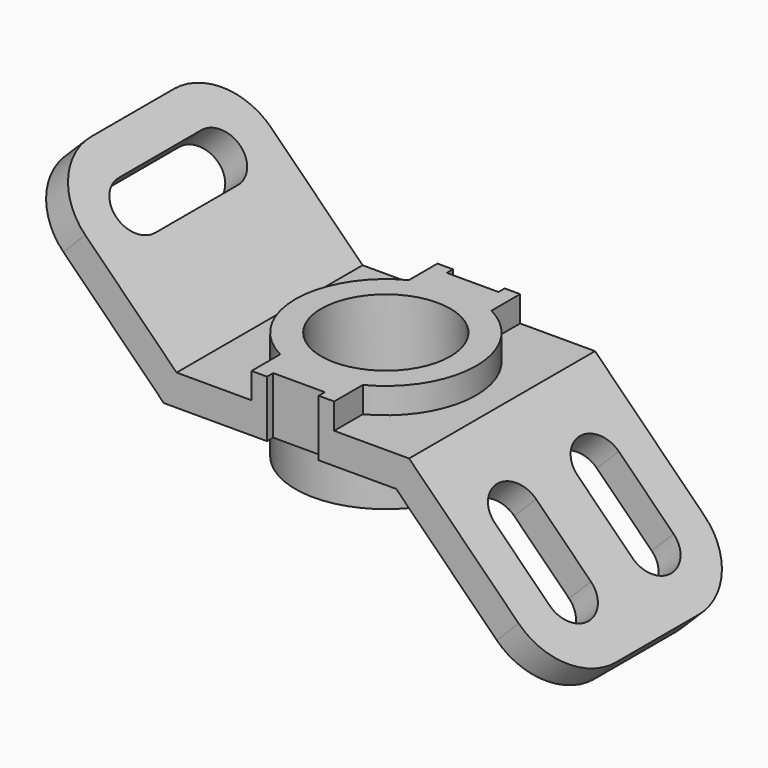
from build123d import *

# Parameters (mm, degrees)
F1_DEPTH       = 45
F2_R           = 35
F3_DEPTH       = 10
F4_R           = 35
F5_DEPTH       = 20
F9_D           = 25
F9_CBORE_D     = 50
F9_CBORE_DEPTH = 32
F10_W          = 20
F10_H          = 3
F11_DEPTH      = 78.5903577751
F12_R          = 25
F14_DEPTH      = 12
F16_DEPTH      = 12


# Not quite as in the source:
# - a pattern or mirror of a feature is missing from the dataset's text; its kind, count and spacing are read off the source's solid


with BuildPart() as f1:
    # F0 (on Front) → F1 (new body, symmetric)
    with BuildSketch(Plane.XZ):
        Polygon((-45, 0), (-98.033008589, 53.033008589), (-106.5182899632, 44.5477272148), (-49.9705627485, -12), (40.0294372515, -12), (96.6187950266, -68.5893577751), (105.1040764009, -60.1040764009), (45, 0), align=None)
    extrude(amount=F1_DEPTH, both=True)

    # F2 (on face) → F3 (join)
    with BuildSketch(Plane.XY):
        Circle(F2_R)
    extrude(amount=F3_DEPTH)

    # F4 (on face) → F5 (join)
    with BuildSketch(Plane(origin=(0, 0, -12), x_dir=(1, 0, 0), z_dir=(0, 0, -1))):
        Circle(F4_R)
    extrude(amount=F5_DEPTH)

    # F6 (on face) → F7 (join, up to the next surface of F1)
    with BuildSketch(Plane.XZ.offset(45)):
        Polygon((-16, 0), (0, 0), (16, 0), (16, 10), (0, 10), (-16, 10), align=None)
    f7 = extrude(until=Until.NEXT, dir=(0, 1, 0))

    # F7_copies: F7 across plane
    add(f7.mirror(Plane.ZX))

    # F9 (through all)
    with Locations(Plane.XY.offset(10)):
        with Locations((0, 0)):
            CounterBoreHole(F9_D / 2, F9_CBORE_D / 2, F9_CBORE_DEPTH)

    # F10 (on face) → F11 (cut, through all)
    with BuildSketch(Plane.XY.offset(10)):
        with Locations((0, 43.5)):
            Rectangle(F10_W, F10_H)
    f11 = extrude(amount=-F11_DEPTH, mode=Mode.SUBTRACT)

    # F11_copies: F11 across plane
    add(f11.mirror(Plane(origin=(0, 0, 0), x_dir=(0, 0, -1), z_dir=(0, -1, 0))), mode=Mode.SUBTRACT)

    # F12
    f12_edges = [f1.edges().sort_by_distance(p)[0] for p in [
        (-102.275649, -45, 48.790368),
        (-102.275649, 45, 48.790368),
        (100.861436, -45, -64.346717),
        (100.861436, 45, -64.346717),
    ]]
    fillet(f12_edges, radius=F12_R)

    # F13 (on face) → F14 (cut, through all)
    with BuildSketch(Plane(origin=(-22.5, 0, -22.5), x_dir=(0, 1, 0), z_dir=(0.7071067812, 0, 0.7071067812))):
        with BuildLine():
            Line((20, 91.8198051534), (-20, 91.8198051534))
            ThreePointArc((-20, 91.8198051534), (-30, 81.8198051534), (-20, 71.8198051534))
            Line((-20, 71.8198051534), (20, 71.8198051534))
            ThreePointArc((20, 71.8198051534), (30, 81.8198051534), (20, 91.8198051534))
        make_face()
    extrude(amount=-F14_DEPTH, mode=Mode.SUBTRACT)

    # F15 (on face) → F16 (cut, through all)
    with BuildSketch(Plane(origin=(22.5, 0, 22.5), x_dir=(0, 1, 0), z_dir=(0.7071067812, 0, 0.7071067812))):
        with BuildLine():
            Line((-30, -61.8198051534), (-30, -91.8198051534))
            ThreePointArc((-30, -91.8198051534), (-20, -101.8198051534), (-10, -91.8198051534))
            Line((-10, -91.8198051534), (-10, -61.8198051534))
            ThreePointArc((-10, -61.8198051534), (-20, -51.8198051534), (-30, -61.8198051534))
        make_face()
    f16 = extrude(amount=-F16_DEPTH, mode=Mode.SUBTRACT)

    # F16_copies: F16 across plane
    add(f16.mirror(Plane.ZX), mode=Mode.SUBTRACT)


solid = f1.part
